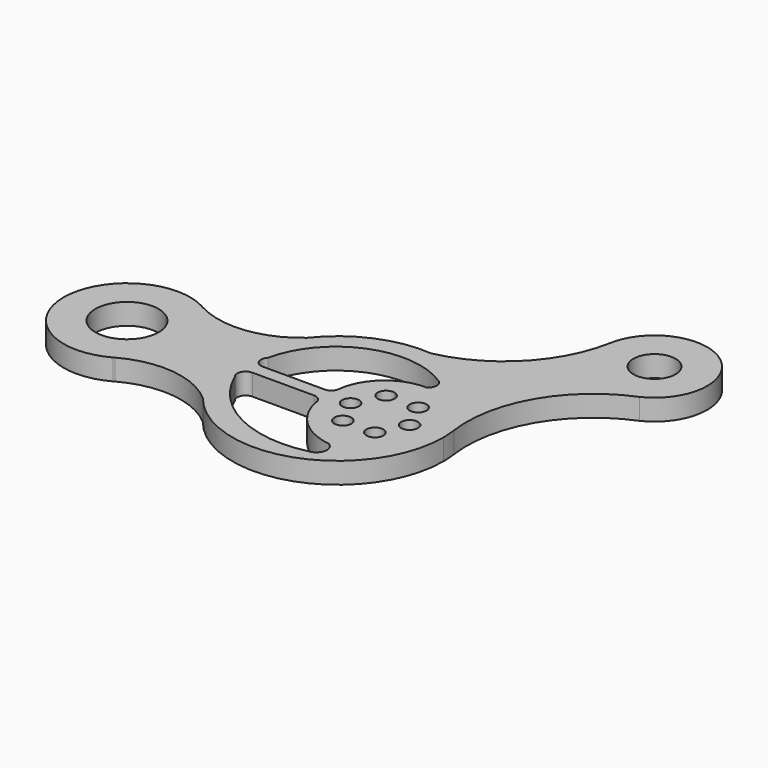
from build123d import *

# Parameters (mm, degrees)
F0_R     = 40
F1_DEPTH = 100


with BuildPart() as f1:
    # F0 (on Top) → F1 (new body)
    with BuildSketch(Plane.XY):
        with BuildLine():
            ThreePointArc((-849.0953685383, -259.2832277711), (-739.9313653682, -149.5470002399), (-700, 0))
            Line((-700, 0), (-850, 0))
            ThreePointArc((-850, 0), (-1000, -150), (-1150, 0))
            Line((-1150, 0), (-1300, 0))
            ThreePointArc((-1300, 0), (-1153.2850393406, -257.8831066867), (-856.6420219043, -263.5308143582))
            ThreePointArc((-856.6420219043, -263.5308143582), (-852.8801904642, -261.3865975578), (-849.0953685383, -259.2832277711))
        make_face()
        with BuildLine():
            ThreePointArc((-849.0953685383, 259.2832277711), (-739.9313653682, 149.5470002399), (-700, 0))
            Line((-700, 0), (-500, 0))
            ThreePointArc((-500, 0), (-472.4467242206, 163.6890123778), (-392.8236289072, 309.3373507551))
            ThreePointArc((-392.8236289072, 309.3373507551), (-613.0653910459, 212.3510174227), (-849.0953685383, 259.2832277711))
        make_face()
        with BuildLine():
            Line((-850, 0), (-700, 0))
            ThreePointArc((-700, 0), (-739.9313653682, 149.5470002399), (-849.0953685383, 259.2832277711))
            ThreePointArc((-849.0953685383, 259.2832277711), (-852.8801904642, 261.3865975578), (-856.6420219043, 263.5308143582))
            ThreePointArc((-856.6420219043, 263.5308143582), (-1153.2850393406, 257.8831066867), (-1300, 0))
            Line((-1300, 0), (-1150, 0))
            ThreePointArc((-1150, 0), (-1000, 150), (-850, 0))
        make_face()
        with BuildLine():
            Line((-500, 0), (-700, 0))
            ThreePointArc((-700, 0), (-739.9313653682, -149.5470002399), (-849.0953685383, -259.2832277711))
            ThreePointArc((-849.0953685383, -259.2832277711), (-613.0653910459, -212.3510174227), (-392.8236289072, -309.3373507551))
            ThreePointArc((-392.8236289072, -309.3373507551), (-472.4467242206, -163.6890123778), (-500, 0))
        make_face()
        with BuildLine():
            ThreePointArc((-392.8236289072, 309.3373507551), (-472.4467242206, 163.6890123778), (-500, 0))
            Line((-500, 0), (-20, 0))
            ThreePointArc((-20, 0), (36.5716696241, 147.2792613729), (177.1925530051, 218.8145798652))
            Line((177.1925530051, 218.8145798652), (314.6601955249, 388.5729807285))
            ThreePointArc((314.6601955249, 388.5729807285), (187.4065310938, 463.5502045123), (43.7997133909, 498.0778906023))
            ThreePointArc((43.7997133909, 498.0778906023), (-198.3939798634, 458.9551489568), (-392.8236289072, 309.3373507551))
        make_face()
        with BuildLine():
            ThreePointArc((-406.6148611623, 92.9051428836), (-169.1586966122, 377.4272459242), (200, 344.8678553104))
            ThreePointArc((200, 344.8678553104), (221.7006400578, 309.2991411686), (200, 273.7304270267))
            ThreePointArc((200, 273.7304270267), (37.9889182283, 215.8833684246), (-43.9509044765, 64.6228704059))
            ThreePointArc((-43.9509044765, 64.6228704059), (-56.0926702606, 37.1503028891), (-83.9313566685, 25.8732473601))
            Line((-83.9313566685, 25.8732473601), (-377.1313636694, 25.8732473601))
            ThreePointArc((-377.1313636694, 25.8732473601), (-413.7460862611, 49.7685247754), (-406.6148611623, 92.9051428836))
        make_face(mode=Mode.SUBTRACT)
        with BuildLine():
            Line((-20, 0), (-500, 0))
            ThreePointArc((-500, 0), (-472.4467242206, -163.6890123778), (-392.8236289072, -309.3373507551))
            ThreePointArc((-392.8236289072, -309.3373507551), (163.6890123778, -472.4467242206), (500, 0))
            ThreePointArc((500, 0), (498.8554636471, 33.8116309782), (495.4270944424, 67.4684673932))
            ThreePointArc((495.4270944424, 67.4684673932), (495.2295651607, 68.8764953304), (495.0353730255, 70.2849873978))
            ThreePointArc((495.0353730255, 70.2849873978), (435.0040690697, 246.5186806164), (314.6601955249, 388.5729807285))
            Line((314.6601955249, 388.5729807285), (177.1925530051, 218.8145798652))
            ThreePointArc((177.1925530051, 218.8145798652), (347.2792613729, 163.4283303759), (420, 0))
            ThreePointArc((420, 0), (200, -220), (-20, 0))
        make_face()
        with BuildLine():
            ThreePointArc((-406.6148611623, -102.8346635677), (-413.7460862611, -59.6980454595), (-377.1313636694, -35.8027680442))
            Line((-377.1313636694, -35.8027680442), (-83.9313566685, -35.8027680442))
            ThreePointArc((-83.9313566685, -35.8027680442), (-55.2084121975, -47.9640816364), (-43.9509044765, -77.0531449985))
            ThreePointArc((-43.9509044765, -77.0531449985), (41.5727461521, -229.7491196269), (200, -304.1208933235))
            ThreePointArc((200, -304.1208933235), (225.7915227703, -357.1958613892), (182.8680932522, -397.6894915104))
            ThreePointArc((182.8680932522, -397.6894915104), (-165.7061110263, -357.8861419627), (-406.6148611623, -102.8346635677))
        make_face(mode=Mode.SUBTRACT)
        with BuildLine():
            ThreePointArc((177.1925530051, 218.8145798652), (36.5716696241, 147.2792613729), (-20, 0))
            Line((-20, 0), (0, 0))
            Line((0, 0), (89.7600051949, 110.8443751857))
            ThreePointArc((89.7600051949, 110.8443751857), (94.1057606724, 154.5806536289), (135.9827631274, 167.9247275238))
            Line((135.9827631274, 167.9247275238), (177.1925530051, 218.8145798652))
        make_face()
        with BuildLine():
            Line((0, 0), (-20, 0))
            ThreePointArc((-20, 0), (200, -220), (420, 0))
            ThreePointArc((420, 0), (347.2792613729, 163.4283303759), (177.1925530051, 218.8145798652))
            Line((177.1925530051, 218.8145798652), (135.9827631274, 167.9247275238))
            ThreePointArc((135.9827631274, 167.9247275238), (157.0635818103, 153.5775860217), (165.1915991306, 129.4078379869))
            ThreePointArc((165.1915991306, 129.4078379869), (134.750266469, 90.5667273088), (89.7600051949, 110.8443751857))
            Line((89.7600051949, 110.8443751857), (0, 0))
        make_face()
        with Locations((125.1915991306, -127.0277351141)):
            Circle(F0_R, mode=Mode.SUBTRACT)
        with Locations((277.0611941814, -127.0277351141)):
            Circle(F0_R, mode=Mode.SUBTRACT)
        with BuildLine():
            ThreePointArc((100, 0), (60, -40), (20, 0))
            ThreePointArc((20, 0), (60, 40), (100, 0))
        make_face(mode=Mode.SUBTRACT)
        with Locations((340, 0)):
            Circle(F0_R, mode=Mode.SUBTRACT)
        with Locations((277.0611941814, 129.4078379869)):
            Circle(F0_R, mode=Mode.SUBTRACT)
        with BuildLine():
            ThreePointArc((508.4647709692, 972.9408629012), (347.8579835974, 665.3239807328), (43.7997133909, 498.0778906023))
            ThreePointArc((43.7997133909, 498.0778906023), (187.4065310938, 463.5502045123), (314.6601955249, 388.5729807285))
            Line((314.6601955249, 388.5729807285), (597.8543714973, 738.2886633841))
            ThreePointArc((597.8543714973, 738.2886633841), (521.5619679737, 843.5778116935), (508.4647709692, 972.9408629012))
        make_face()
        with BuildLine():
            Line((597.8543714973, 738.2886633841), (314.6601955249, 388.5729807285))
            ThreePointArc((314.6601955249, 388.5729807285), (435.0040690697, 246.5186806164), (495.0353730255, 70.2849873978))
            ThreePointArc((495.0353730255, 70.2849873978), (564.4809221518, 441.9510892686), (842.4187636125, 698.2886242833))
            ThreePointArc((842.4187636125, 698.2886242833), (714.8315735034, 685.8533594049), (597.8543714973, 738.2886633841))
        make_face()
        with BuildLine():
            ThreePointArc((1005.1844692598, 932.5751537484), (775.4338572426, 1181.7537288433), (508.4647709692, 972.9408629012))
            ThreePointArc((508.4647709692, 972.9408629012), (521.5619679737, 843.5778116935), (597.8543714973, 738.2886633841))
            ThreePointArc((597.8543714973, 738.2886633841), (714.8315735034, 685.8533594049), (842.4187636125, 698.2886242833))
            ThreePointArc((842.4187636125, 698.2886242833), (853.4019929681, 703.1204808996), (864.4796509854, 707.7317343393))
            ThreePointArc((864.4796509854, 707.7317343393), (967.1087428004, 799.9550109182), (1005.1844692598, 932.5751537484))
        make_face()
        with BuildLine():
            ThreePointArc((855.1844692598, 932.5751537484), (798.2355789406, 842.3166253134), (692.2524301548, 854.8605576027))
            ThreePointArc((692.2524301548, 854.8605576027), (677.4698731141, 995.5071928533), (818.1165083648, 1010.2897498941))
            ThreePointArc((818.1165083648, 1010.2897498941), (845.4429976948, 975.6262634292), (855.1844692598, 932.5751537484))
        make_face(mode=Mode.SUBTRACT)
    extrude(amount=F1_DEPTH)


solid = f1.part
